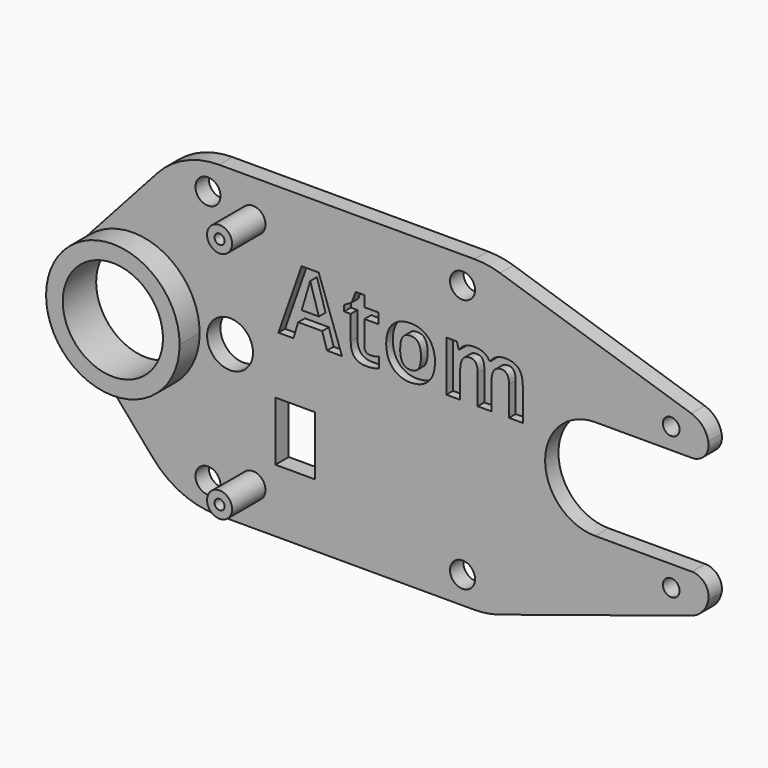
from build123d import *

# Parameters (mm, degrees)
F0_R          = 1.5
F0_R_2        = 1
F0_R_3        = 2.75
F1_DEPTH      = 2
F2_DEPTH      = 5
F3_R          = 10
F4_R          = 10
F5_R          = 10
F6_R          = 10
F7_R          = 3
F8_R          = 2
F9_R          = 3
F10_R         = 2
F11_R         = 1.5
F11_R_2       = 0.6
F12_DEPTH     = 5
F13_W         = 4.7696251422
F13_H         = 7.0821696427
F14_DEPTH     = 2
F15_TEXT_SIZE = 11.0484520658
F16_DEPTH     = 1


# Not quite as in the source:
# - Text() gives the source's letters only with a copy of the font that has no kerning and outlines rounded to 1/6400 em; it was checked with that copy


with BuildPart() as f1:
    # F0 (on Front) → F1 (new body)
    with BuildSketch(Plane.XZ):
        with BuildLine():
            Line((-26.0642077774, -18.5), (10.9590468556, -18.5))
            Line((10.9590468556, -18.5), (37.5, -10))
            Line((37.5, -10), (37.5, -6))
            Line((37.5, -6), (23.8934811205, -6))
            ThreePointArc((23.8934811205, -6), (17.8934811205, 0), (23.8934811205, 6))
            Line((23.8934811205, 6), (37.5, 6))
            Line((37.5, 6), (37.5, 10))
            Line((37.5, 10), (11.0067082752, 18.5))
            Line((11.0067082752, 18.5), (-25.6080199033, 18.5))
            Line((-25.6080199033, 18.5), (-37.3901407018, 5.4135240382))
            ThreePointArc((-37.3901407018, 5.4135240382), (-28.5949290555, 7.4538958141), (-23.5, 0))
            ThreePointArc((-23.5, 0), (-28.6715728753, -7.4833147735), (-37.5, -5.2915026221))
            Line((-37.5, -5.2915026221), (-37.5, -5.2920114501))
            Line((-37.5, -5.2920114501), (-26.0642077774, -18.5))
        make_face()
        with Locations((-22.5, -15.25)):
            Circle(F0_R, mode=Mode.SUBTRACT)
        with Locations((8, -15.25)):
            Circle(F0_R, mode=Mode.SUBTRACT)
        with Locations((33, -8.5)):
            Circle(F0_R_2, mode=Mode.SUBTRACT)
        with Locations((-19.8600627482, 0)):
            Circle(F0_R_3, mode=Mode.SUBTRACT)
        with Locations((-22.5, 15.25)):
            Circle(F0_R, mode=Mode.SUBTRACT)
        with Locations((33, 8.5)):
            Circle(F0_R_2, mode=Mode.SUBTRACT)
        with Locations((8, 15.25)):
            Circle(F0_R, mode=Mode.SUBTRACT)
    extrude(amount=F1_DEPTH)

    # F0 (on Front) → F2 (join)
    with BuildSketch(Plane.XZ):
        with BuildLine():
            Line((-37.5, 0), (-37.5, -5.2915026221))
            ThreePointArc((-37.5, -5.2915026221), (-28.6715728753, -7.4833147735), (-23.5, 0))
            ThreePointArc((-23.5, 0), (-28.5949290555, 7.4538958141), (-37.3901407018, 5.4135240382))
            Line((-37.3901407018, 5.4135240382), (-37.5, 5.2915026221))
            Line((-37.5, 5.2915026221), (-37.5, 0))
        make_face()
        with BuildLine():
            ThreePointArc((-25.5, 0), (-31.5, -6), (-37.5, 0))
            ThreePointArc((-37.5, 0), (-31.5, 6), (-25.5, 0))
        make_face(mode=Mode.SUBTRACT)
        with BuildLine():
            ThreePointArc((-37.5, 5.2915026221), (-39.5, 0), (-37.5, -5.2915026221))
            Line((-37.5, -5.2915026221), (-37.5, 0))
            Line((-37.5, 0), (-37.5, 5.2915026221))
        make_face()
    extrude(amount=F2_DEPTH)

    # F3
    f3_edges = [f1.edges().sort_by_distance(p)[0] for p in [
        (-25.60802, -1, 18.5),
    ]]
    fillet(f3_edges, radius=F3_R)

    # F4
    f4_edges = [f1.edges().sort_by_distance(p)[0] for p in [
        (11.006708, -1, 18.5),
    ]]
    fillet(f4_edges, radius=F4_R)

    # F5
    f5_edges = [f1.edges().sort_by_distance(p)[0] for p in [
        (-26.064208, -1, -18.5),
    ]]
    fillet(f5_edges, radius=F5_R)

    # F6
    f6_edges = [f1.edges().sort_by_distance(p)[0] for p in [
        (10.959047, -1, -18.5),
    ]]
    fillet(f6_edges, radius=F6_R)

    # F7
    f7_edges = [f1.edges().sort_by_distance(p)[0] for p in [
        (37.5, -1, -10),
    ]]
    fillet(f7_edges, radius=F7_R)

    # F8
    f8_edges = [f1.edges().sort_by_distance(p)[0] for p in [
        (37.5, -1, -6),
    ]]
    fillet(f8_edges, radius=F8_R)

    # F9
    f9_edges = [f1.edges().sort_by_distance(p)[0] for p in [
        (37.5, -1, 10),
    ]]
    fillet(f9_edges, radius=F9_R)

    # F10
    f10_edges = [f1.edges().sort_by_distance(p)[0] for p in [
        (37.5, -1, 6),
    ]]
    fillet(f10_edges, radius=F10_R)

    # F11 (on face) → F12 (join)
    with BuildSketch(Plane.XZ.offset(2)):
        with Locations((-17.1100627482, 14)):
            Circle(F11_R)
        with Locations((-17.1100627482, 14)):
            Circle(F11_R_2, mode=Mode.SUBTRACT)
        with Locations((-17.1100627482, -14)):
            Circle(F11_R)
        with Locations((-17.1100627482, -14)):
            Circle(F11_R_2, mode=Mode.SUBTRACT)
    extrude(amount=F12_DEPTH)

    # F13 (on face) → F14 (cut)
    with BuildSketch(Plane.XZ.offset(2)):
        with Locations((-12.0383864269, -7.4053445132)):
            Rectangle(F13_W, F13_H)
    extrude(amount=-F14_DEPTH, mode=Mode.SUBTRACT)

    # F15 (on face) → F16 (cut)
    with BuildSketch(Plane.XZ.offset(2)):
        with Locations((-14.0641518301, 3.0975750016)):
            Text('Atom', F15_TEXT_SIZE, font='Open Sans', font_style=FontStyle.BOLD, text_align=(TextAlign.LEFT, TextAlign.BOTTOM))
    extrude(amount=-F16_DEPTH, mode=Mode.SUBTRACT)


solid = f1.part
